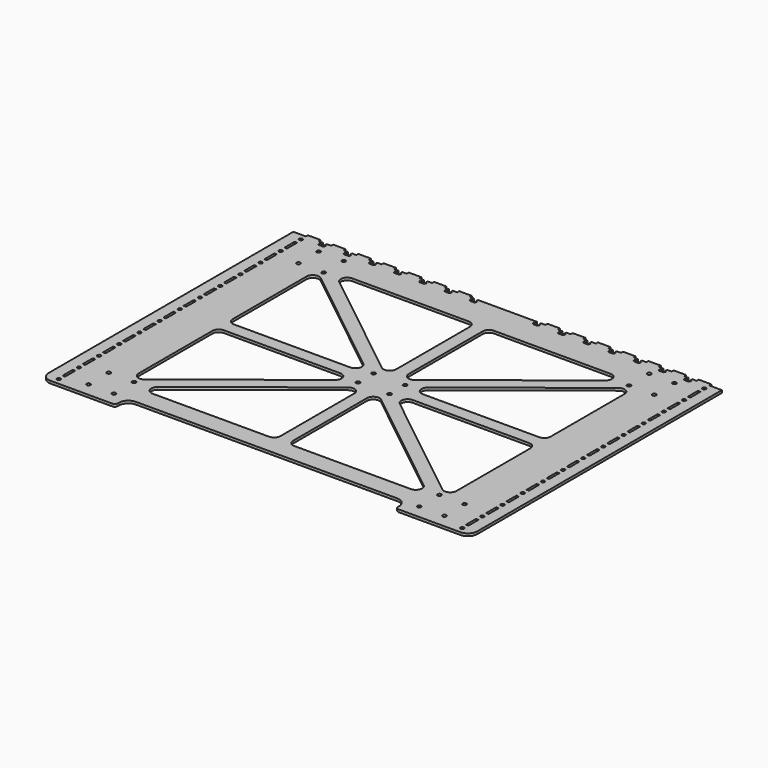
from build123d import *

# Parameters (mm, degrees)
F0_R     = 2.75
F0_W     = 4
F0_H     = 20
F0_R_2   = 3
F1_DEPTH = 4


# Not quite as in the source:
# - a feature names something its author has since deleted; it is built from what else it names


with BuildPart() as f1:
    # F0 (on Top) → F1 (new body)
    with BuildSketch(Plane.XY):
        with BuildLine():
            Line((-320, 250), (-340, 250))
            Line((-340, 250), (-340, -235))
            ThreePointArc((-340, -235), (-335.6066017178, -245.6066017178), (-325, -250))
            Line((-325, -250), (-262.25, -250))
            Line((-262.25, -250), (-227.25, -250))
            ThreePointArc((-227.25, -250), (-223.7144660941, -248.5355339059), (-222.25, -245))
            Line((-222.25, -245), (-222.25, -243))
            ThreePointArc((-222.25, -243), (-217.8566017178, -232.3933982822), (-207.25, -228))
            Line((-207.25, -228), (207.25, -228))
            ThreePointArc((207.25, -228), (217.8566017178, -232.3933982822), (222.25, -243))
            Line((222.25, -243), (222.25, -245))
            ThreePointArc((222.25, -245), (223.7144660941, -248.5355339059), (227.25, -250))
            Line((227.25, -250), (325, -250))
            ThreePointArc((325, -250), (335.6066017178, -245.6066017178), (340, -235))
            Line((340, -235), (340, 250))
            Line((340, 250), (320, 250))
            Line((320, 250), (320, 254))
            Line((320, 254), (300, 254))
            Line((300, 254), (300, 250))
            Line((300, 250), (293, 250))
            Line((293, 250), (293, 246))
            Line((293, 246), (295, 246))
            Line((295, 246), (295, 243.6))
            Line((295, 243.6), (293.4, 242))
            Line((293.4, 242), (290, 242))
            Line((290, 242), (286.6, 242))
            Line((286.6, 242), (285, 243.6))
            Line((285, 243.6), (285, 246))
            Line((285, 246), (287, 246))
            Line((287, 246), (287, 250))
            Line((287, 250), (280, 250))
            Line((280, 250), (280, 254))
            Line((280, 254), (260, 254))
            Line((260, 254), (260, 250))
            Line((260, 250), (253, 250))
            Line((253, 250), (253, 246))
            Line((253, 246), (255, 246))
            Line((255, 246), (255, 243.6))
            Line((255, 243.6), (253.4, 242))
            Line((253.4, 242), (250, 242))
            Line((250, 242), (246.6, 242))
            Line((246.6, 242), (245, 243.6))
            Line((245, 243.6), (245, 246))
            Line((245, 246), (247, 246))
            Line((247, 246), (247, 250))
            Line((247, 250), (240, 250))
            Line((240, 250), (240, 254))
            Line((240, 254), (220, 254))
            Line((220, 254), (220, 250))
            Line((220, 250), (213, 250))
            Line((213, 250), (213, 246))
            Line((213, 246), (215, 246))
            Line((215, 246), (215, 243.6))
            Line((215, 243.6), (213.4, 242))
            Line((213.4, 242), (210, 242))
            Line((210, 242), (206.6, 242))
            Line((206.6, 242), (205, 243.6))
            Line((205, 243.6), (205, 246))
            Line((205, 246), (207, 246))
            Line((207, 246), (207, 250))
            Line((207, 250), (200, 250))
            Line((200, 250), (200, 254))
            Line((200, 254), (180, 254))
            Line((180, 254), (180, 250))
            Line((180, 250), (173, 250))
            Line((173, 250), (173, 246))
            Line((173, 246), (175, 246))
            Line((175, 246), (175, 243.6))
            Line((175, 243.6), (173.4, 242))
            Line((173.4, 242), (170, 242))
            Line((170, 242), (166.6, 242))
            Line((166.6, 242), (165, 243.6))
            Line((165, 243.6), (165, 246))
            Line((165, 246), (167, 246))
            Line((167, 246), (167, 250))
            Line((167, 250), (160, 250))
            Line((160, 250), (160, 254))
            Line((160, 254), (140, 254))
            Line((140, 254), (140, 250))
            Line((140, 250), (133, 250))
            Line((133, 250), (133, 246))
            Line((133, 246), (135, 246))
            Line((135, 246), (135, 243.6))
            Line((135, 243.6), (133.4, 242))
            Line((133.4, 242), (130, 242))
            Line((130, 242), (126.6, 242))
            Line((126.6, 242), (125, 243.6))
            Line((125, 243.6), (125, 246))
            Line((125, 246), (127, 246))
            Line((127, 246), (127, 250))
            Line((127, 250), (120, 250))
            Line((120, 250), (120, 254))
            Line((120, 254), (100, 254))
            Line((100, 254), (100, 250))
            Line((100, 250), (93, 250))
            Line((93, 250), (93, 246))
            Line((93, 246), (95, 246))
            Line((95, 246), (95, 243.6))
            Line((95, 243.6), (93.4, 242))
            Line((93.4, 242), (90, 242))
            Line((90, 242), (86.6, 242))
            Line((86.6, 242), (85, 243.6))
            Line((85, 243.6), (85, 246))
            Line((85, 246), (87, 246))
            Line((87, 246), (87, 250))
            Line((87, 250), (80, 250))
            Line((80, 250), (80, 254))
            Line((80, 254), (60, 254))
            Line((60, 254), (60, 250))
            Line((60, 250), (53, 250))
            Line((53, 250), (53, 246))
            Line((53, 246), (55, 246))
            Line((55, 246), (55, 243.6))
            Line((55, 243.6), (53.4, 242))
            Line((53.4, 242), (50, 242))
            Line((50, 242), (46.6, 242))
            Line((46.6, 242), (45, 243.6))
            Line((45, 243.6), (45, 246))
            Line((45, 246), (47, 246))
            Line((47, 246), (47, 250))
            Line((47, 250), (40, 250))
            Line((40, 250), (-40, 250))
            Line((-40, 250), (-47, 250))
            Line((-47, 250), (-47, 246))
            Line((-47, 246), (-45, 246))
            Line((-45, 246), (-45, 243.6))
            Line((-45, 243.6), (-46.6, 242))
            Line((-46.6, 242), (-50, 242))
            Line((-50, 242), (-53.4, 242))
            Line((-53.4, 242), (-55, 243.6))
            Line((-55, 243.6), (-55, 246))
            Line((-55, 246), (-53, 246))
            Line((-53, 246), (-53, 250))
            Line((-53, 250), (-60, 250))
            Line((-60, 250), (-60, 254))
            Line((-60, 254), (-80, 254))
            Line((-80, 254), (-80, 250))
            Line((-80, 250), (-87, 250))
            Line((-87, 250), (-87, 246))
            Line((-87, 246), (-85, 246))
            Line((-85, 246), (-85, 243.6))
            Line((-85, 243.6), (-86.6, 242))
            Line((-86.6, 242), (-90, 242))
            Line((-90, 242), (-93.4, 242))
            Line((-93.4, 242), (-95, 243.6))
            Line((-95, 243.6), (-95, 246))
            Line((-95, 246), (-93, 246))
            Line((-93, 246), (-93, 250))
            Line((-93, 250), (-100, 250))
            Line((-100, 250), (-100, 254))
            Line((-100, 254), (-120, 254))
            Line((-120, 254), (-120, 250))
            Line((-120, 250), (-127, 250))
            Line((-127, 250), (-127, 246))
            Line((-127, 246), (-125, 246))
            Line((-125, 246), (-125, 243.6))
            Line((-125, 243.6), (-126.6, 242))
            Line((-126.6, 242), (-130, 242))
            Line((-130, 242), (-133.4, 242))
            Line((-133.4, 242), (-135, 243.6))
            Line((-135, 243.6), (-135, 246))
            Line((-135, 246), (-133, 246))
            Line((-133, 246), (-133, 250))
            Line((-133, 250), (-140, 250))
            Line((-140, 250), (-140, 254))
            Line((-140, 254), (-160, 254))
            Line((-160, 254), (-160, 250))
            Line((-160, 250), (-167, 250))
            Line((-167, 250), (-167, 246))
            Line((-167, 246), (-165, 246))
            Line((-165, 246), (-165, 243.6))
            Line((-165, 243.6), (-166.6, 242))
            Line((-166.6, 242), (-170, 242))
            Line((-170, 242), (-173.4, 242))
            Line((-173.4, 242), (-175, 243.6))
            Line((-175, 243.6), (-175, 246))
            Line((-175, 246), (-173, 246))
            Line((-173, 246), (-173, 250))
            Line((-173, 250), (-180, 250))
            Line((-180, 250), (-180, 254))
            Line((-180, 254), (-200, 254))
            Line((-200, 254), (-200, 250))
            Line((-200, 250), (-207, 250))
            Line((-207, 250), (-207, 246))
            Line((-207, 246), (-205, 246))
            Line((-205, 246), (-205, 243.6))
            Line((-205, 243.6), (-206.6, 242))
            Line((-206.6, 242), (-210, 242))
            Line((-210, 242), (-213.4, 242))
            Line((-213.4, 242), (-215, 243.6))
            Line((-215, 243.6), (-215, 246))
            Line((-215, 246), (-213, 246))
            Line((-213, 246), (-213, 250))
            Line((-213, 250), (-220, 250))
            Line((-220, 250), (-220, 254))
            Line((-220, 254), (-240, 254))
            Line((-240, 254), (-240, 250))
            Line((-240, 250), (-247, 250))
            Line((-247, 250), (-247, 246))
            Line((-247, 246), (-245, 246))
            Line((-245, 246), (-245, 243.6))
            Line((-245, 243.6), (-246.6, 242))
            Line((-246.6, 242), (-250, 242))
            Line((-250, 242), (-253.4, 242))
            Line((-253.4, 242), (-255, 243.6))
            Line((-255, 243.6), (-255, 246))
            Line((-255, 246), (-253, 246))
            Line((-253, 246), (-253, 250))
            Line((-253, 250), (-260, 250))
            Line((-260, 250), (-260, 254))
            Line((-260, 254), (-280, 254))
            Line((-280, 254), (-280, 250))
            Line((-280, 250), (-287, 250))
            Line((-287, 250), (-287, 246))
            Line((-287, 246), (-285, 246))
            Line((-285, 246), (-285, 243.6))
            Line((-285, 243.6), (-286.6, 242))
            Line((-286.6, 242), (-290, 242))
            Line((-290, 242), (-293.4, 242))
            Line((-293.4, 242), (-295, 243.6))
            Line((-295, 243.6), (-295, 246))
            Line((-295, 246), (-293, 246))
            Line((-293, 246), (-293, 250))
            Line((-293, 250), (-300, 250))
            Line((-300, 250), (-300, 254))
            Line((-300, 254), (-320, 254))
            Line((-320, 254), (-320, 250))
        make_face()
        with Locations((-320, -240)):
            Circle(F0_R, mode=Mode.SUBTRACT)
        with Locations((-320, -220)):
            Rectangle(F0_W, F0_H, mode=Mode.SUBTRACT)
        with Locations((-282.25, -228)):
            Circle(F0_R_2, mode=Mode.SUBTRACT)
        with Locations((-320, -200)):
            Circle(F0_R, mode=Mode.SUBTRACT)
        with Locations((-282.25, -188)):
            Circle(F0_R_2, mode=Mode.SUBTRACT)
        with Locations((-242.25, -228)):
            Circle(F0_R_2, mode=Mode.SUBTRACT)
        with Locations((-242.25, -188)):
            Circle(F0_R_2, mode=Mode.SUBTRACT)
        with Locations((-320, -180)):
            Rectangle(F0_W, F0_H, mode=Mode.SUBTRACT)
        with Locations((-320, -160)):
            Circle(F0_R, mode=Mode.SUBTRACT)
        with Locations((-320, -140)):
            Rectangle(F0_W, F0_H, mode=Mode.SUBTRACT)
        with Locations((-320, -120)):
            Circle(F0_R, mode=Mode.SUBTRACT)
        with Locations((-320, -100)):
            Rectangle(F0_W, F0_H, mode=Mode.SUBTRACT)
        with Locations((-320, -80)):
            Circle(F0_R, mode=Mode.SUBTRACT)
        with Locations((-320, -60)):
            Rectangle(F0_W, F0_H, mode=Mode.SUBTRACT)
        with Locations((-320, -40)):
            Circle(F0_R, mode=Mode.SUBTRACT)
        with Locations((-320, -20)):
            Rectangle(F0_W, F0_H, mode=Mode.SUBTRACT)
        with Locations((-320, 0)):
            Circle(F0_R, mode=Mode.SUBTRACT)
        with BuildLine():
            ThreePointArc((-252.25, -20), (-249.3210678119, -12.9289321881), (-242.25, -10))
            Line((-242.25, -10), (-57.4011890671, -10))
            ThreePointArc((-57.4011890671, -10), (-47.9579768489, -16.709750313), (-51.187083858, -27.8348513994))
            Line((-51.187083858, -27.8348513994), (-236.0358947909, -174.4451571155))
            ThreePointArc((-236.0358947909, -174.4451571155), (-246.6008015301, -175.6142229772), (-252.25, -166.6103057161))
            Line((-252.25, -166.6103057161), (-252.25, -20))
        make_face(mode=Mode.SUBTRACT)
        with BuildLine():
            Line((-211.062916142, -180.1651486006), (-26.2141052091, -33.5548428845))
            ThreePointArc((-26.2141052091, -33.5548428845), (-15.6491984699, -32.3857770228), (-10, -41.3896942839))
            Line((-10, -41.3896942839), (-10, -188))
            ThreePointArc((-10, -188), (-12.9289321881, -195.0710678119), (-20, -198))
            Line((-20, -198), (-204.8488109329, -198))
            ThreePointArc((-204.8488109329, -198), (-214.2920231511, -191.290249687), (-211.062916142, -180.1651486006))
        make_face(mode=Mode.SUBTRACT)
        with Locations((-25, -15.5)):
            Circle(F0_R_2, mode=Mode.SUBTRACT)
        with Locations((242.25, -228)):
            Circle(F0_R_2, mode=Mode.SUBTRACT)
        with Locations((242.25, -188)):
            Circle(F0_R_2, mode=Mode.SUBTRACT)
        with Locations((282.25, -228)):
            Circle(F0_R_2, mode=Mode.SUBTRACT)
        with Locations((320, -240)):
            Circle(F0_R, mode=Mode.SUBTRACT)
        with Locations((320, -220)):
            Rectangle(F0_W, F0_H, mode=Mode.SUBTRACT)
        with Locations((282.25, -188)):
            Circle(F0_R_2, mode=Mode.SUBTRACT)
        with Locations((320, -200)):
            Circle(F0_R, mode=Mode.SUBTRACT)
        with Locations((320, -180)):
            Rectangle(F0_W, F0_H, mode=Mode.SUBTRACT)
        with Locations((320, -160)):
            Circle(F0_R, mode=Mode.SUBTRACT)
        with Locations((320, -140)):
            Rectangle(F0_W, F0_H, mode=Mode.SUBTRACT)
        with BuildLine():
            ThreePointArc((20, -198), (12.9289321881, -195.0710678119), (10, -188))
            Line((10, -188), (10, -41.3896942839))
            ThreePointArc((10, -41.3896942839), (15.6491984699, -32.3857770228), (26.2141052091, -33.5548428845))
            Line((26.2141052091, -33.5548428845), (211.062916142, -180.1651486006))
            ThreePointArc((211.062916142, -180.1651486006), (214.2920231511, -191.290249687), (204.8488109329, -198))
            Line((204.8488109329, -198), (20, -198))
        make_face(mode=Mode.SUBTRACT)
        with BuildLine():
            Line((236.0358947909, -174.4451571155), (51.187083858, -27.8348513994))
            ThreePointArc((51.187083858, -27.8348513994), (47.9579768489, -16.709750313), (57.4011890671, -10))
            Line((57.4011890671, -10), (242.25, -10))
            ThreePointArc((242.25, -10), (249.3210678119, -12.9289321881), (252.25, -20))
            Line((252.25, -20), (252.25, -166.6103057161))
            ThreePointArc((252.25, -166.6103057161), (246.6008015301, -175.6142229772), (236.0358947909, -174.4451571155))
        make_face(mode=Mode.SUBTRACT)
        with Locations((25, -15.5)):
            Circle(F0_R_2, mode=Mode.SUBTRACT)
        with Locations((320, -120)):
            Circle(F0_R, mode=Mode.SUBTRACT)
        with Locations((320, -100)):
            Rectangle(F0_W, F0_H, mode=Mode.SUBTRACT)
        with Locations((320, -80)):
            Circle(F0_R, mode=Mode.SUBTRACT)
        with Locations((320, -60)):
            Rectangle(F0_W, F0_H, mode=Mode.SUBTRACT)
        with Locations((320, -40)):
            Circle(F0_R, mode=Mode.SUBTRACT)
        with Locations((320, -20)):
            Rectangle(F0_W, F0_H, mode=Mode.SUBTRACT)
        with Locations((320, 0)):
            Circle(F0_R, mode=Mode.SUBTRACT)
        with Locations((-320, 20)):
            Rectangle(F0_W, F0_H, mode=Mode.SUBTRACT)
        with Locations((-320, 40)):
            Circle(F0_R, mode=Mode.SUBTRACT)
        with Locations((-320, 60)):
            Rectangle(F0_W, F0_H, mode=Mode.SUBTRACT)
        with Locations((-320, 80)):
            Circle(F0_R, mode=Mode.SUBTRACT)
        with Locations((-320, 100)):
            Rectangle(F0_W, F0_H, mode=Mode.SUBTRACT)
        with Locations((-320, 120)):
            Circle(F0_R, mode=Mode.SUBTRACT)
        with Locations((-25, 15.5)):
            Circle(F0_R_2, mode=Mode.SUBTRACT)
        with BuildLine():
            Line((-57.4011890671, 10), (-242.25, 10))
            ThreePointArc((-242.25, 10), (-249.3210678119, 12.9289321881), (-252.25, 20))
            Line((-252.25, 20), (-252.25, 166.6103057161))
            ThreePointArc((-252.25, 166.6103057161), (-246.6008015301, 175.6142229772), (-236.0358947909, 174.4451571155))
            Line((-236.0358947909, 174.4451571155), (-51.187083858, 27.8348513994))
            ThreePointArc((-51.187083858, 27.8348513994), (-47.9579768489, 16.709750313), (-57.4011890671, 10))
        make_face(mode=Mode.SUBTRACT)
        with BuildLine():
            ThreePointArc((-10, 41.3896942839), (-15.6491984699, 32.3857770228), (-26.2141052091, 33.5548428845))
            Line((-26.2141052091, 33.5548428845), (-211.062916142, 180.1651486006))
            ThreePointArc((-211.062916142, 180.1651486006), (-214.2920231511, 191.290249687), (-204.8488109329, 198))
            Line((-204.8488109329, 198), (-20, 198))
            ThreePointArc((-20, 198), (-12.9289321881, 195.0710678119), (-10, 188))
            Line((-10, 188), (-10, 41.3896942839))
        make_face(mode=Mode.SUBTRACT)
        with Locations((-320, 140)):
            Rectangle(F0_W, F0_H, mode=Mode.SUBTRACT)
        with Locations((-320, 160)):
            Circle(F0_R, mode=Mode.SUBTRACT)
        with Locations((-320, 180)):
            Rectangle(F0_W, F0_H, mode=Mode.SUBTRACT)
        with Locations((-282.25, 188)):
            Circle(F0_R_2, mode=Mode.SUBTRACT)
        with Locations((-242.25, 188)):
            Circle(F0_R_2, mode=Mode.SUBTRACT)
        with Locations((-320, 200)):
            Circle(F0_R, mode=Mode.SUBTRACT)
        with Locations((-320, 220)):
            Rectangle(F0_W, F0_H, mode=Mode.SUBTRACT)
        with Locations((-320, 240)):
            Circle(F0_R, mode=Mode.SUBTRACT)
        with Locations((-282.25, 228)):
            Circle(F0_R_2, mode=Mode.SUBTRACT)
        with Locations((-242.25, 228)):
            Circle(F0_R_2, mode=Mode.SUBTRACT)
        with Locations((25, 15.5)):
            Circle(F0_R_2, mode=Mode.SUBTRACT)
        with BuildLine():
            ThreePointArc((57.4011890671, 10), (47.9579768489, 16.709750313), (51.187083858, 27.8348513994))
            Line((51.187083858, 27.8348513994), (236.0358947909, 174.4451571155))
            ThreePointArc((236.0358947909, 174.4451571155), (246.6008015301, 175.6142229772), (252.25, 166.6103057161))
            Line((252.25, 166.6103057161), (252.25, 20))
            ThreePointArc((252.25, 20), (249.3210678119, 12.9289321881), (242.25, 10))
            Line((242.25, 10), (57.4011890671, 10))
        make_face(mode=Mode.SUBTRACT)
        with BuildLine():
            ThreePointArc((26.2141052091, 33.5548428845), (15.6491984699, 32.3857770228), (10, 41.3896942839))
            Line((10, 41.3896942839), (10, 188))
            ThreePointArc((10, 188), (12.9289321881, 195.0710678119), (20, 198))
            Line((20, 198), (204.8488109329, 198))
            ThreePointArc((204.8488109329, 198), (214.2920231511, 191.290249687), (211.062916142, 180.1651486006))
            Line((211.062916142, 180.1651486006), (26.2141052091, 33.5548428845))
        make_face(mode=Mode.SUBTRACT)
        with Locations((320, 20)):
            Rectangle(F0_W, F0_H, mode=Mode.SUBTRACT)
        with Locations((320, 40)):
            Circle(F0_R, mode=Mode.SUBTRACT)
        with Locations((320, 60)):
            Rectangle(F0_W, F0_H, mode=Mode.SUBTRACT)
        with Locations((320, 80)):
            Circle(F0_R, mode=Mode.SUBTRACT)
        with Locations((320, 100)):
            Rectangle(F0_W, F0_H, mode=Mode.SUBTRACT)
        with Locations((320, 120)):
            Circle(F0_R, mode=Mode.SUBTRACT)
        with Locations((242.25, 188)):
            Circle(F0_R_2, mode=Mode.SUBTRACT)
        with Locations((320, 140)):
            Rectangle(F0_W, F0_H, mode=Mode.SUBTRACT)
        with Locations((282.25, 188)):
            Circle(F0_R_2, mode=Mode.SUBTRACT)
        with Locations((320, 160)):
            Circle(F0_R, mode=Mode.SUBTRACT)
        with Locations((320, 180)):
            Rectangle(F0_W, F0_H, mode=Mode.SUBTRACT)
        with Locations((242.25, 228)):
            Circle(F0_R_2, mode=Mode.SUBTRACT)
        with Locations((320, 200)):
            Circle(F0_R, mode=Mode.SUBTRACT)
        with Locations((320, 220)):
            Rectangle(F0_W, F0_H, mode=Mode.SUBTRACT)
        with Locations((282.25, 228)):
            Circle(F0_R_2, mode=Mode.SUBTRACT)
        with Locations((320, 240)):
            Circle(F0_R, mode=Mode.SUBTRACT)
    extrude(amount=F1_DEPTH)


solid = f1.part
